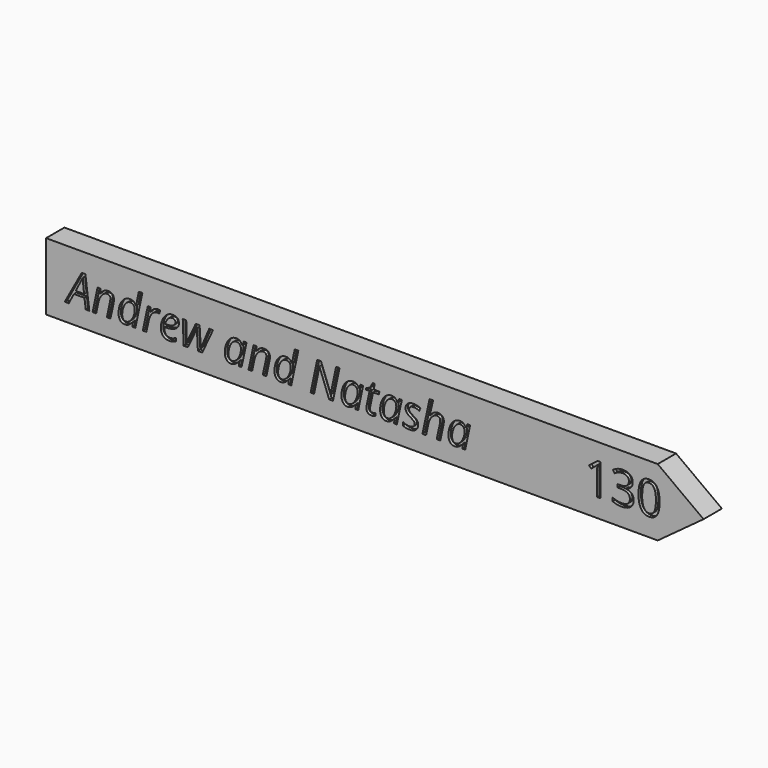
from build123d import *

# Parameters (mm, degrees)
F1_DEPTH       = 15
F2_TEXT_SIZE   = 28.4468884476
F2_TEXT_SIZE_2 = 29.2940065265
F3_DEPTH       = 2


# Not quite as in the source:
# - Text() gives the source's letters only with a copy of the font that has no kerning and outlines rounded to 1/6400 em; it was checked with that copy


with BuildPart() as f1:
    # F0 (on Front) → F1 (new body)
    with BuildSketch(Plane.XZ):
        Polygon((0, 44), (0, 0), (400, 0), (430, 22), (400, 44), align=None)
    extrude(amount=F1_DEPTH)

    # F2 (on face) → F3 (cut)
    with BuildSketch(Plane.XZ.offset(15)):
        with Locations((13.8236023486, 11.3039752468)):
            Text('Andrew and Natasha', F2_TEXT_SIZE, font='Open Sans', font_style=FontStyle.ITALIC, text_align=(TextAlign.LEFT, TextAlign.BOTTOM))
        with Locations((352.4820087478, 12.1125690639)):
            Text('130', F2_TEXT_SIZE_2, font='Open Sans', text_align=(TextAlign.LEFT, TextAlign.BOTTOM))
    extrude(amount=-F3_DEPTH, mode=Mode.SUBTRACT)


solid = f1.part
